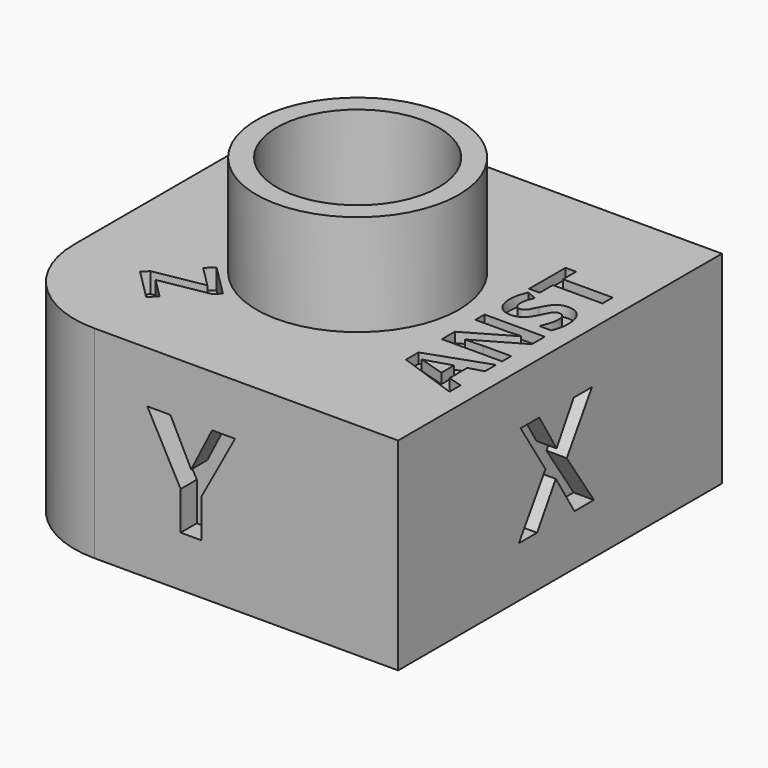
from build123d import *

# Parameters (mm, degrees)
F0_W          = 20
F0_H          = 20
F1_DEPTH      = 10
F2_R          = 5
F2_R_2        = 4
F3_DEPTH      = 5
F4_TEXT_SIZE  = 13.8888888889
F5_DEPTH      = 2
F6_TEXT_SIZE  = 6.9444444444
F7_DEPTH      = 1
F8_TEXT_SIZE  = 6.9444444444
F9_DEPTH      = 1
F10_R         = 5
F11_TEXT_SIZE = 4.1666666667
F12_DEPTH     = 1
F13_TEXT_SIZE = 4.1666666667
F14_DEPTH     = 0.5
F16_DEPTH     = 5


# Not quite as in the source:
# - Text() gives the source's letters only with a copy of the font that has no kerning and outlines rounded to 1/6400 em; it was checked with that copy


with BuildPart() as f1:
    # F0 (on Top) → F1 (new body)
    with BuildSketch(Plane.XY):
        with Locations((10, 10)):
            Rectangle(F0_W, F0_H)
    extrude(amount=F1_DEPTH)

    # F2 (on face) → F3 (join)
    with BuildSketch(Plane.XY.offset(10)):
        with Locations((10, 10)):
            Circle(F2_R)
        with Locations((10, 10)):
            Circle(F2_R_2, mode=Mode.SUBTRACT)
    extrude(amount=F3_DEPTH)

    # F4 (on face) → F5 (cut)
    with BuildSketch(Plane(origin=(0, 0, 0), x_dir=(1, 0, 0), z_dir=(0, 0, -1))):
        with Locations((5.8637152778, -15)):
            Text('Z', F4_TEXT_SIZE, font='Open Sans', text_align=(TextAlign.LEFT, TextAlign.BOTTOM))
    extrude(amount=-F5_DEPTH, mode=Mode.SUBTRACT)

    # F6 (on face) → F7 (cut)
    with BuildSketch(Plane.XZ):
        with Locations((7.6079644097, 2.5)):
            Text('Y', F6_TEXT_SIZE, font='Open Sans', font_style=FontStyle.BOLD, text_align=(TextAlign.LEFT, TextAlign.BOTTOM))
    extrude(amount=-F7_DEPTH, mode=Mode.SUBTRACT)

    # F8 (on face) → F9 (cut)
    with BuildSketch(Plane.YZ.offset(20)):
        with Locations((7.4587673611, 2.5)):
            Text('X', F8_TEXT_SIZE, font='Open Sans', font_style=FontStyle.BOLD, text_align=(TextAlign.LEFT, TextAlign.BOTTOM))
    extrude(amount=-F9_DEPTH, mode=Mode.SUBTRACT)

    # F10
    f10_edges = [f1.edges().sort_by_distance(p)[0] for p in [
        (0, 0, 5),
    ]]
    fillet(f10_edges, radius=F10_R)

    # F11 (on face) → F12 (cut)
    with BuildSketch(Plane.XY.offset(10)):
        with Locations(Location((7.1213203436, 5.2946278255), (0, 0, 135))):
            Text('Z', F11_TEXT_SIZE, font='Open Sans', font_style=FontStyle.BOLD, text_align=(TextAlign.LEFT, TextAlign.BOTTOM))
    extrude(amount=-F12_DEPTH, mode=Mode.SUBTRACT)

    # F13 (on face) → F14 (cut)
    with BuildSketch(Plane.XY.offset(10)):
        with Locations(Location((19, 4.4215494792), (0, 0, 90))):
            Text('ANST', F13_TEXT_SIZE, font='Open Sans', font_style=FontStyle.BOLD, text_align=(TextAlign.LEFT, TextAlign.BOTTOM))
    extrude(amount=-F14_DEPTH, mode=Mode.SUBTRACT)

    # F15 (on face) → F16 (cut)
    with BuildSketch(Plane.XY.offset(10)):
        Polygon((11.7320508076, 13), (8.2679491924, 13), (6.5358983849, 10), (8.2679491924, 7), (11.7320508076, 7), (13.4641016151, 10), align=None)
    extrude(amount=-F16_DEPTH, mode=Mode.SUBTRACT)


solid = f1.part
